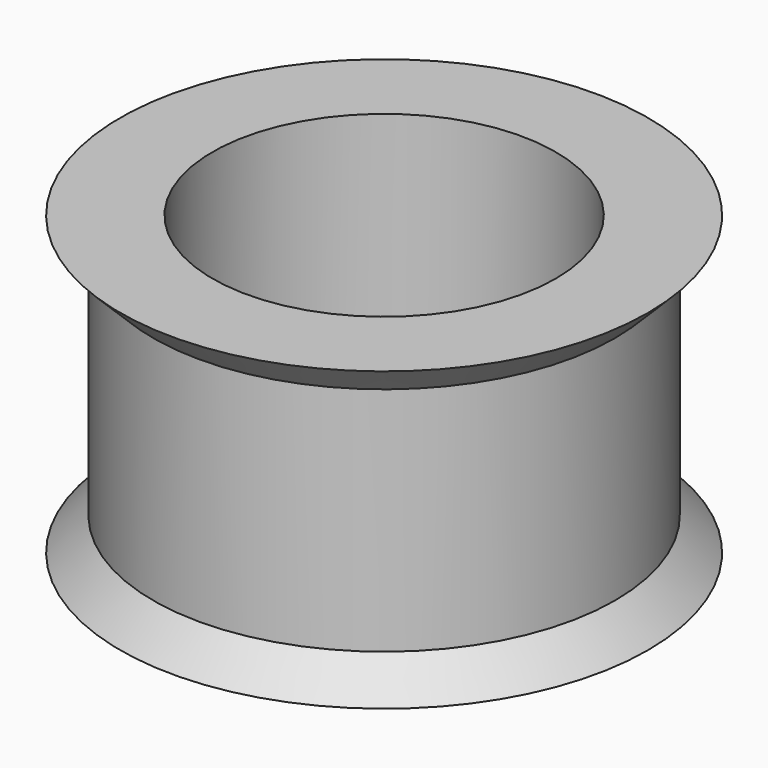
from build123d import *

# Parameters (mm, degrees)
F0_R     = 7
F0_R_2   = 5.2
F1_DEPTH = 9
F0_R_3   = 8
F2_DEPTH = 1
F3_R     = 8
F3_R_2   = 7
F4_DEPTH = 1
F5_SIZE  = 0.99999


# Not quite as in the source:
# - a fillet or chamfer is up to 0.001 mm smaller than in the source, because OpenCascade refuses the exact size


with BuildPart() as f1:
    # F0 (on Top) → F1 (new body)
    with BuildSketch(Plane.XY):
        Circle(F0_R)
        Circle(F0_R_2, mode=Mode.SUBTRACT)
    extrude(amount=F1_DEPTH)

    # F0 (on Top) → F2 (join)
    with BuildSketch(Plane.XY):
        Circle(F0_R_3)
        Circle(F0_R, mode=Mode.SUBTRACT)
    extrude(amount=F2_DEPTH)

    # F3 (on face) → F4 (join)
    with BuildSketch(Plane.XY.offset(9)):
        Circle(F3_R)
        Circle(F3_R_2, mode=Mode.SUBTRACT)
    extrude(amount=-F4_DEPTH)

    # F5 (size 1 in the source; OpenCascade refuses exactly that, so slightly less here)
    f5_edges = [f1.edges().sort_by_distance(p)[0] for p in [
        (-8, 0, 8),
        (-8, 0, 1),
    ]]
    chamfer(f5_edges, length=F5_SIZE)


solid = f1.part
